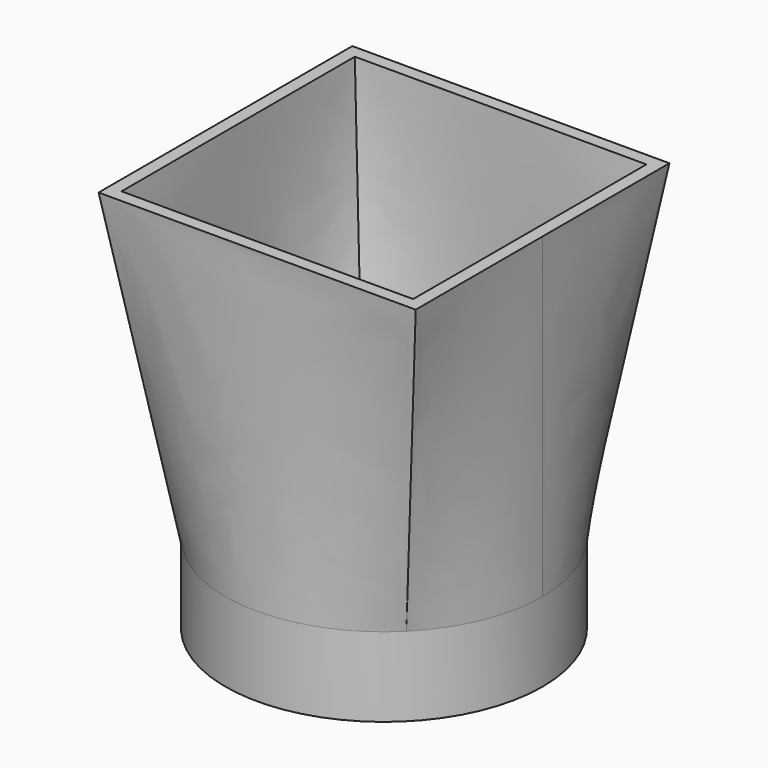
from build123d import *

# Parameters (mm, degrees)
F0_R     = 20
F2_W     = 40
F2_H     = 40
F4_T     = 1.6
F5_DEPTH = 10


# Not quite as in the source:
# - a shell that OpenCascade refuses in one call is made with other operations: the cavity is built on its own and cut out


with BuildPart() as f3:
    # F0 (on Top) → F3 section 0
    with BuildSketch(Plane.XY):
        Circle(F0_R)
    # F2 (on offset) → F3 section 1
    with BuildSketch(Plane.XY.offset(40)):
        Rectangle(F2_W, F2_H)
    loft()

    # F4: shell of thickness 1.6, made by hand


with BuildPart() as f4_core1:
    # F4_t2: copy of F3
    add(f3.part)

    # the walls: a layer under each face that stays
    f4_faces = [f4_core1.faces().sort_by_distance(p)[0] for p in [
        (19.2387953231, 8.8268343228, 20),
        (0, 19.9999999992, 20),
        (-19.9999999992, 0, 20),
        (0, -19.9999999992, 20),
        (19.2387953231, -8.8268343228, 20),
        (0, 0, 0),
    ]]
    thicken(f4_faces, amount=-F4_T, mode=Mode.SUBTRACT)


with BuildPart() as f3_1:
    add(f3.part)

    # what is left inside the walls is the cavity
    f4_cavity = [f4_core1.part.solids().sort_by_distance(p)[0] for p in [
        (3.677504, 7.355008, 39.984),
    ]]
    add(f4_cavity, mode=Mode.SUBTRACT)

    # F0 (on Top) → F5 (join)
    with BuildSketch(Plane.XY):
        Circle(F0_R)
    extrude(amount=-F5_DEPTH)


solid = f3_1.part
